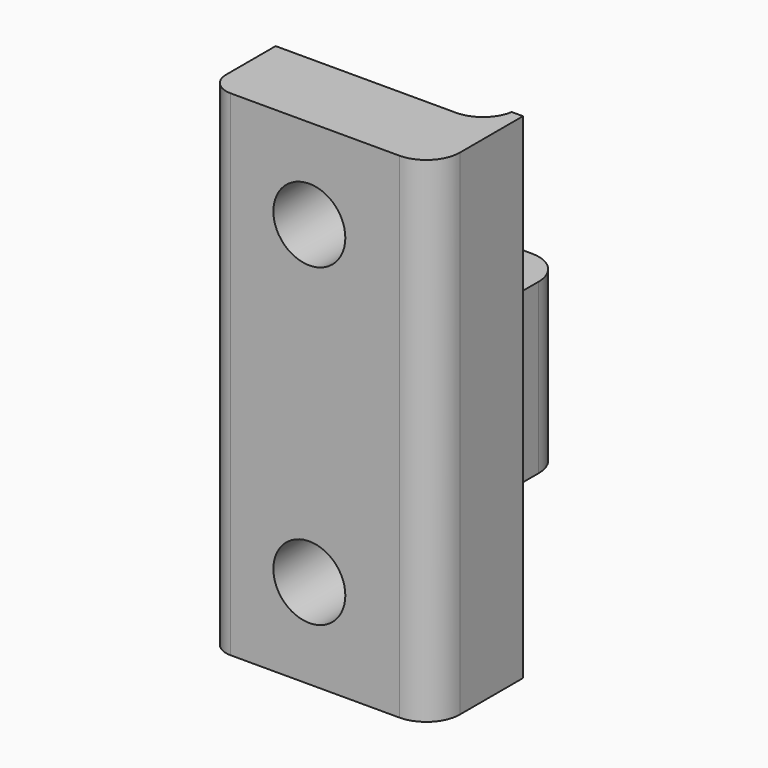
from build123d import *

# Parameters (mm, degrees)
F0_W        = 10
F0_H        = 22
F1_DEPTH    = 5
F2_W        = 9.5
F2_H        = 1.25
F3_DEPTH    = 22
F4_R        = 1.5
F5_R        = 1.6
F6_DEPTH    = 3.75
F7_W        = 9.5
F7_H        = 7.5
F8_DEPTH    = 4.25
F9_T1_DEPTH = 10.9475498644
F9_T3_DEPTH = 10.9475498644
F9_T5_DEPTH = 15
F9_T7_DEPTH = 15
F10_R       = 1


# Not quite as in the source:
# - a fillet or chamfer that OpenCascade refuses, or shapes differently, is made with other operations: its cross-section is extruded or revolved along the edge and cut away or added


with BuildPart() as f1:
    # F0 (on Front) → F1 (new body)
    with BuildSketch(Plane.XZ):
        with Locations((-1, 0)):
            Rectangle(F0_W, F0_H)
    extrude(amount=F1_DEPTH)

    # F2 (on face) → F3 (cut, through all)
    with BuildSketch(Plane(origin=(0, 0, -11), x_dir=(1, 0, 0), z_dir=(0, 0, -1))):
        with Locations((-1.25, 0.625)):
            Rectangle(F2_W, F2_H)
    extrude(amount=-F3_DEPTH, mode=Mode.SUBTRACT)

    # F4
    f4_edges = [f1.edges().sort_by_distance(p)[0] for p in [
        (4, -5, 0),
    ]]
    fillet(f4_edges, radius=F4_R)

    # F5 (on face) → F6 (cut, through all)
    with BuildSketch(Plane.XZ.offset(5)):
        with Locations((-1.5, 7)):
            Circle(F5_R)
        with Locations((-1.5, -7)):
            Circle(F5_R)
    extrude(amount=-F6_DEPTH, mode=Mode.SUBTRACT)

    # F7 (on face) → F8 (join)
    with BuildSketch(Plane(origin=(0, -1.25, 0), x_dir=(-1, 0, 0), z_dir=(0, 1, 0))):
        with Locations((1.25, 0)):
            Rectangle(F7_W, F7_H)
    extrude(amount=F8_DEPTH)

    # F9: fillet of radius 1.5 on 4 edges, made by hand

    # F9_s2 → F9_t1 (join)
    with BuildSketch(Plane.XY.offset(0.0524501356)):
        with BuildLine():
            ThreePointArc((2.0209800542, -1.25), (2.9892258908, -0.8956439237), (3.5, 0))
            Line((3.5, 0), (3.5, -1.25))
            Line((3.5, -1.25), (2.0209800542, -1.25))
        make_face()
    extrude(amount=F9_T1_DEPTH)

    # F9_s4 → F9_t3 (join)
    with BuildSketch(Plane.XY.offset(-11)):
        with BuildLine():
            ThreePointArc((2.0209800542, -1.25), (2.9892258908, -0.8956439237), (3.5, 0))
            Line((3.5, 0), (3.5, -1.25))
            Line((3.5, -1.25), (2.0209800542, -1.25))
        make_face()
    extrude(amount=F9_T3_DEPTH)

    # F9_s6 → F9_t5 (cut)
    with BuildSketch(Plane.XY.offset(-7.5)):
        with BuildLine():
            ThreePointArc((-4.5, 3), (-5.5606601718, 2.5606601718), (-6, 1.5))
            Line((-6, 1.5), (-6, 3))
            Line((-6, 3), (-4.5, 3))
        make_face()
    extrude(amount=F9_T5_DEPTH, mode=Mode.SUBTRACT)

    # F9_s8 → F9_t7 (cut)
    with BuildSketch(Plane.XY.offset(-7.5)):
        with BuildLine():
            ThreePointArc((3.5, 1.5), (3.0606601718, 2.5606601718), (2, 3))
            Line((2, 3), (3.5, 3))
            Line((3.5, 3), (3.5, 1.5))
        make_face()
    extrude(amount=F9_T7_DEPTH, mode=Mode.SUBTRACT)

    # F10
    f10_edges = [f1.edges().sort_by_distance(p)[0] for p in [
        (-6, -5, 0),
    ]]
    fillet(f10_edges, radius=F10_R)


solid = f1.part
